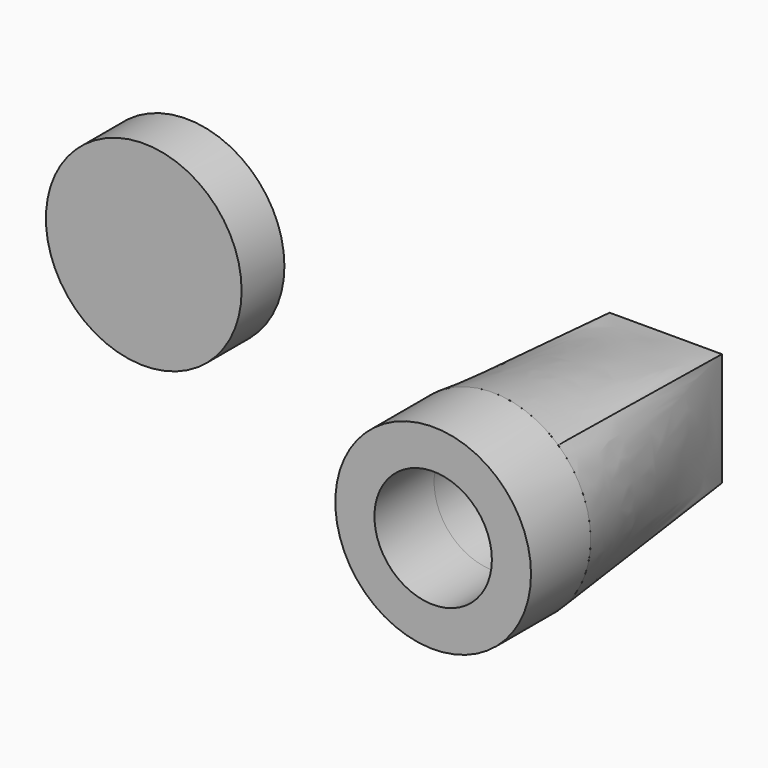
from build123d import *

# Parameters (mm, degrees)
F0_R          = 25.4
F1_DEPTH      = 76.2
F2_W          = 59.7524605691
F2_H          = 58.5865583271
F3_DEPTH      = 43.434
F3_DEPTH_BACK = 30.226
F4_W          = 29.1475430131
F4_H          = 29.4390162453
F6_R          = 15.24
F7_DEPTH      = 59.69
F8_R          = 25.4
F9_DEPTH      = 101.6
F10_W         = 93.4799709357
F10_H         = 55.210987106
F11_DEPTH     = 89.916


# Not quite as in the source:
# - the arcs of a loft's sections are written as splines that run evenly, so that the points pair up as in the source's solid


with BuildPart() as f1:
    # F0 (on Front) → F1 (new body)
    with BuildSketch(Plane.XZ):
        Circle(F0_R)
    extrude(amount=F1_DEPTH)

    # F2 (on Right) → F3 (cut, two sides)
    with BuildSketch(Plane.YZ) as f3_sk:
        with Locations((-26.9614737481, -0.2914750949)):
            Rectangle(F2_W, F2_H)
    extrude(amount=-F3_DEPTH, mode=Mode.SUBTRACT)
    extrude(f3_sk.sketch, amount=F3_DEPTH_BACK, mode=Mode.SUBTRACT)


with BuildPart() as f5:
    # F3_face (on face) → F5 section 0
    with BuildSketch(Plane(origin=(0, -56.8377040327, 0), x_dir=(-1, 0, 0), z_dir=(0, 1, 0))):
        with BuildLine():
            add(Edge.make_bspline(
                [(-16.9623986454, 18.9060051887), (-18.1997937915, 17.7958187934), (-19.3278172281, 16.5637900788), (-21.321881876, 13.9032734939), (-22.18787378, 12.4748514101), (-23.6245819975, 9.4764331911), (-24.1952627855, 7.9065111976), (-25.0194026816, 4.6854188751), (-25.2728414111, 3.0343281939), (-25.4527417517, -0.2856534605), (-25.3791989144, -1.9544623407), (-24.9079462304, -5.2457482939), (-24.5102480363, -6.8681439836), (-23.405952304, -10.0042519622), (-22.6993820716, -11.5178867049), (-21.0044807567, -14.3782978381), (-20.0161915839, -15.7250034994), (-18.9060051887, -16.9623986454)],
                knots=[0, 0, 0, 0, 0.125, 0.125, 0.25, 0.25, 0.375, 0.375, 0.5, 0.5, 0.625, 0.625, 0.75, 0.75, 0.875, 0.875, 1, 1, 1, 1], degree=3))
            add(Edge.make_bspline(
                [(-18.9060051887, -16.9623986454), (-17.7958187934, -18.1997937915), (-16.5637900788, -19.3278172281), (-13.9032734939, -21.321881876), (-12.4748514101, -22.18787378), (-9.4764331911, -23.6245819975), (-7.9065111976, -24.1952627855), (-4.6854188751, -25.0194026816), (-3.0343281939, -25.2728414111), (0.2856534605, -25.4527417517), (1.9544623407, -25.3791989144), (5.2457482939, -24.9079462304), (6.8681439836, -24.5102480363), (10.0042519622, -23.405952304), (11.5178867049, -22.6993820716), (14.3782978381, -21.0044807567), (15.7250034994, -20.0161915839), (16.9623986454, -18.9060051887)],
                knots=[0, 0, 0, 0, 0.125, 0.125, 0.25, 0.25, 0.375, 0.375, 0.5, 0.5, 0.625, 0.625, 0.75, 0.75, 0.875, 0.875, 1, 1, 1, 1], degree=3))
            add(Edge.make_bspline(
                [(16.9623986454, -18.9060051887), (18.1997937915, -17.7958187934), (19.3278172281, -16.5637900788), (21.321881876, -13.9032734939), (22.18787378, -12.4748514101), (23.6245819975, -9.4764331911), (24.1952627855, -7.9065111976), (25.0194026816, -4.6854188751), (25.2728414111, -3.0343281939), (25.4527417517, 0.2856534605), (25.3791989144, 1.9544623407), (24.9079462304, 5.2457482939), (24.5102480363, 6.8681439836), (23.405952304, 10.0042519622), (22.6993820716, 11.5178867049), (21.0044807567, 14.3782978381), (20.0161915839, 15.7250034994), (18.9060051887, 16.9623986454)],
                knots=[0, 0, 0, 0, 0.125, 0.125, 0.25, 0.25, 0.375, 0.375, 0.5, 0.5, 0.625, 0.625, 0.75, 0.75, 0.875, 0.875, 1, 1, 1, 1], degree=3))
            add(Edge.make_bspline(
                [(18.9060051887, 16.9623986454), (17.7958187934, 18.1997937915), (16.5637900788, 19.3278172281), (13.9032734939, 21.321881876), (12.4748514101, 22.18787378), (9.4764331911, 23.6245819975), (7.9065111976, 24.1952627855), (4.6854188751, 25.0194026816), (3.0343281939, 25.2728414111), (-0.2856534605, 25.4527417517), (-1.9544623407, 25.3791989144), (-5.2457482939, 24.9079462304), (-6.8681439836, 24.5102480363), (-10.0042519622, 23.405952304), (-11.5178867049, 22.6993820716), (-14.3782978381, 21.0044807567), (-15.7250034994, 20.0161915839), (-16.9623986454, 18.9060051887)],
                knots=[0, 0, 0, 0, 0.125, 0.125, 0.25, 0.25, 0.375, 0.375, 0.5, 0.5, 0.625, 0.625, 0.75, 0.75, 0.875, 0.875, 1, 1, 1, 1], degree=3))
        make_face()
    # F4 (on Front) → F5 section 1
    with BuildSketch(Plane.XZ):
        with Locations((-0.582951121, 0.8744257502)):
            Rectangle(F4_W, F4_H)
    loft(ruled=True)


with BuildPart() as f7_tool:
    # F6 (on face) → F7 (new body)
    with BuildSketch(Plane.XZ.offset(76.2)):
        Circle(F6_R)
    extrude(amount=-F7_DEPTH)


with BuildPart() as f1_1:
    add(f1.part)

    # F7: cut by f7_tool
    add(f7_tool.part, mode=Mode.SUBTRACT)


with BuildPart() as f5_1:
    add(f5.part)

    # F7: cut by f7_tool
    add(f7_tool.part, mode=Mode.SUBTRACT)


with BuildPart() as f9:
    # F8 (on Front) → F9 (new body)
    with BuildSketch(Plane.XZ):
        with Locations((-54.7973774374, 57.2749190032)):
            Circle(F8_R)
    extrude(amount=F9_DEPTH)

    # F10 (on Right) → F11 (cut)
    with BuildSketch(Plane.YZ):
        with Locations((-40.9772868734, 56.4336283132)):
            Rectangle(F10_W, F10_H)
    extrude(amount=-F11_DEPTH, mode=Mode.SUBTRACT)


solid = Compound([f1_1.part, f5_1.part, f9.part])
